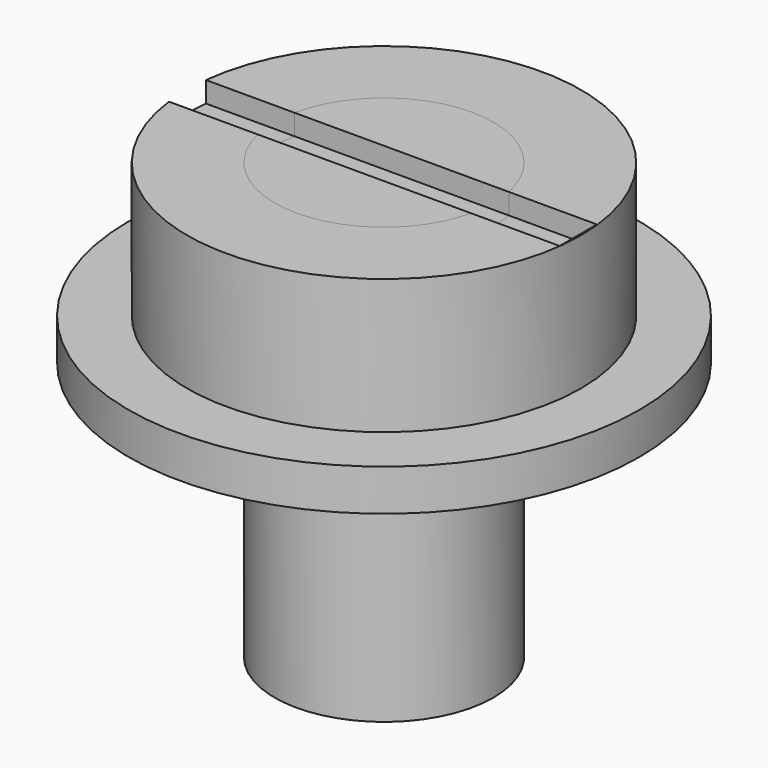
from build123d import *

# Parameters (mm, degrees)
F0_R     = 2.11
F1_DEPTH = 5.8
F2_R     = 4.925
F2_R_2   = 2.11
F3_DEPTH = 0.8
F4_R     = 3.8
F4_R_2   = 2.11
F5_DEPTH = 2.6
F6_R     = 2.11
F7_DEPTH = 2.6
F9_DEPTH = 0.4


with BuildPart() as f1:
    # F0 (on Top) → F1 (new body)
    with BuildSketch(Plane.XY):
        Circle(F0_R)
    extrude(amount=F1_DEPTH)


with BuildPart() as f3:
    # F2 (on face) → F3 (new body)
    with BuildSketch(Plane.XY.offset(5.8)):
        Circle(F2_R)
        Circle(F2_R_2, mode=Mode.SUBTRACT)
    extrude(amount=-F3_DEPTH)

    # F4 (on face) → F5 (join)
    with BuildSketch(Plane.XY.offset(5.8)):
        Circle(F4_R)
        Circle(F4_R_2, mode=Mode.SUBTRACT)
    extrude(amount=F5_DEPTH)


with BuildPart() as f7:
    # F6 (on face) → F7 (new body)
    with BuildSketch(Plane.XY.offset(5.8)):
        Circle(F6_R)
    extrude(amount=F7_DEPTH)


with BuildPart() as f9_tool:
    # F8 (on face) → F9 (new body)
    with BuildSketch(Plane.XY.offset(8.4)):
        with BuildLine():
            Line((-2.0663575468, 0.4269267956), (-3.8097645156, 0.4269267956))
            Line((-3.8097645156, 0.4269267956), (-3.8097645156, -0.4721327277))
            Line((-3.8097645156, -0.4721327277), (-2.0564996201, -0.4721327277))
            ThreePointArc((-2.0564996201, -0.4721327277), (-2.1098731742, -0.0231341469), (-2.0663575468, 0.4269267956))
        make_face()
        with BuildLine():
            Line((2.0663575468, 0.4269267956), (-2.0663575468, 0.4269267956))
            ThreePointArc((-2.0663575468, 0.4269267956), (-2.1098731742, -0.0231341469), (-2.0564996201, -0.4721327277))
            Line((-2.0564996201, -0.4721327277), (2.0564996201, -0.4721327277))
            ThreePointArc((2.0564996201, -0.4721327277), (2.0965822424, -0.2375771471), (2.11, 0))
            ThreePointArc((2.11, 0), (2.099061031, 0.2145758331), (2.0663575468, 0.4269267956))
        make_face()
        with BuildLine():
            Line((3.7648119032, 0.4269267956), (2.0663575468, 0.4269267956))
            ThreePointArc((2.0663575468, 0.4269267956), (2.099061031, 0.2145758331), (2.11, 0))
            ThreePointArc((2.11, 0), (2.0965822424, -0.2375771471), (2.0564996201, -0.4721327277))
            Line((2.0564996201, -0.4721327277), (3.7648119032, -0.4721327277))
            Line((3.7648119032, -0.4721327277), (3.7648119032, 0.4269267956))
        make_face()
    extrude(amount=-F9_DEPTH)


with BuildPart() as f3_1:
    add(f3.part)

    # F9: cut by f9_tool
    add(f9_tool.part, mode=Mode.SUBTRACT)


with BuildPart() as f7_1:
    add(f7.part)

    # F9: cut by f9_tool
    add(f9_tool.part, mode=Mode.SUBTRACT)


solid = Compound([f1.part, f3_1.part, f7_1.part])
